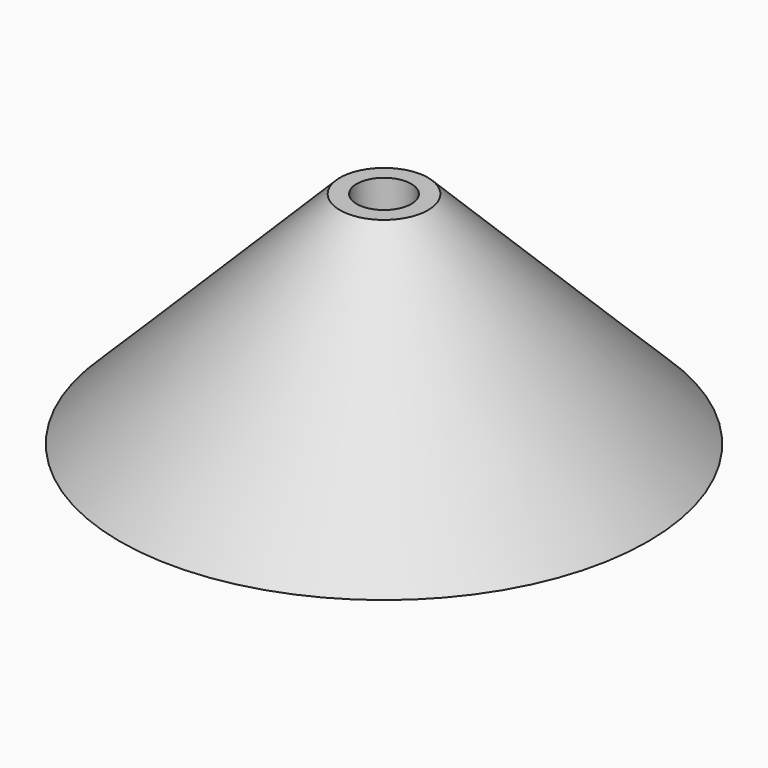
from build123d import *

# Parameters (mm, degrees)
F0_R           = 152.4
F1_DEPTH       = 127
F3_D           = 17.5
F3_CBORE_D     = 31.5
F3_CBORE_DEPTH = 20
F4_SIZE        = 126.99999


# Not quite as in the source:
# - a fillet or chamfer is up to 0.001 mm smaller than in the source, because OpenCascade refuses the exact size


with BuildPart() as f1:
    # F0 (on Top) → F1 (new body)
    with BuildSketch(Plane.XY):
        Circle(F0_R)
    extrude(amount=F1_DEPTH)

    # F3 (through all)
    with Locations(Plane.XY.offset(127)):
        with Locations((0, 0)):
            CounterBoreHole(F3_D / 2, F3_CBORE_D / 2, F3_CBORE_DEPTH)

    # F4 (size 127 in the source; OpenCascade refuses exactly that, so slightly less here)
    f4_edges = [f1.edges().sort_by_distance(p)[0] for p in [
        (-152.4, 0, 127),
    ]]
    chamfer(f4_edges, length=F4_SIZE)


solid = f1.part
